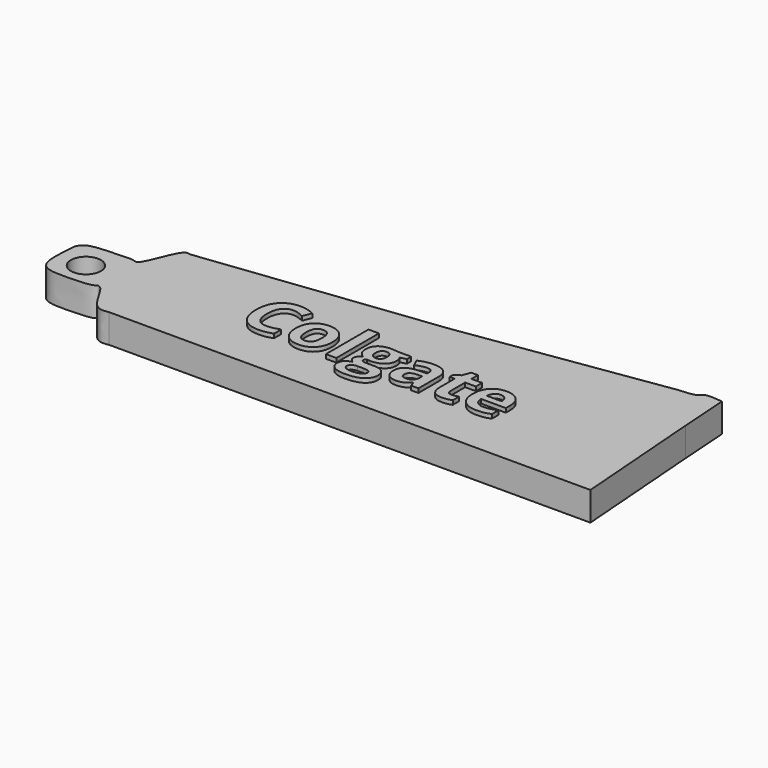
from build123d import *

# Parameters (mm, degrees)
F0_R         = 1.8236553972
F1_DEPTH     = 3.5
F2_TEXT_SIZE = 8.5194750379
F3_DEPTH     = 0.5


# Not quite as in the source:
# - Text() gives the source's letters only with a copy of the font that has no kerning and outlines rounded to 1/6400 em; it was checked with that copy


with BuildPart() as f1:
    # F0 (on Top) → F1 (new body)
    with BuildSketch(Plane.XY):
        with BuildLine():
            add(Edge.make_bspline(
                [(-94.2050293088, 31.265206635), (-94.3971896936, 31.315162363), (-94.9583376122, 31.4610433822), (-95.9054216002, 29.4777531909), (-96.8691566029, 26.8074850092), (-97.4710081074, 26.8823429315), (-97.8983149621, 27.0596648483), (-99.5300476845, 26.9187238719), (-103.2306123724, 26.9127671347), (-103.6583521932, 25.96518302), (-103.8144603372, 25.6193522364)],
                knots=[0, 0, 0, 0, 0.0806326622, 0.235463988, 0.4124921189, 0.4787807152, 0.5456222164, 0.6826832027, 0.8841918992, 1, 1, 1, 1], degree=3))
            add(Edge.make_bspline(
                [(-103.8144603372, 25.6193522364), (-103.9362776366, 24.0968857457), (-104.1299409277, 21.6764916586), (-103.0230108011, 20.2993669542), (-100.4135696071, 20.2585530739), (-97.435923479, 20.4079273263), (-97.2192654941, 20.8016425102), (-96.3493816333, 20.8286988089), (-94.7313642338, 16.8706039662), (-93.3537822149, 17.095992357), (-92.809304595, 17.1850752085)],
                knots=[0, 0, 0, 0, 0.1802033396, 0.2864845305, 0.4344172907, 0.587234469, 0.638819425, 0.7063803162, 0.883949308, 1, 1, 1, 1], degree=3))
            Line((-92.809304595, 17.1850752085), (-47.8415191174, 17.1850752085))
            Line((-47.8415191174, 17.1850752085), (-37.0270833373, 17.1850752085))
            add(Edge.make_bspline(
                [(-37.0270833373, 17.1850752085), (-36.7521914562, 17.1850752085), (-36.0885433471, 17.1850752085), (-34.9738631658, 17.1850752085), (-34.3208983541, 17.1850752085)],
                knots=[0, 0, 0, 0, 0.4142133119, 1, 1, 1, 1], degree=3))
            Line((-34.3208983541, 17.1850752085), (-35.5386808515, 33.149138093))
            Line((-35.5386808515, 33.149138093), (-35.9455570579, 39.1874983907))
            add(Edge.make_bspline(
                [(-35.9455570579, 39.1874983907), (-36.8082930393, 39.2807532353), (-38.1547953916, 39.426299347), (-38.4848889619, 38.553670295), (-39.7685209587, 38.4821076009), (-40.5851490796, 38.4365804493)],
                knots=[0, 0, 0, 0, 0.3935045367, 0.6141563534, 1, 1, 1, 1], degree=3))
            Line((-40.5851490796, 38.4365804493), (-65.6604096293, 34.6819981933))
            Line((-65.6604096293, 34.6819981933), (-94.2050293088, 31.265206635))
        make_face()
        with Locations((-100.5051881075, 23.2916418463)):
            Circle(F0_R, mode=Mode.SUBTRACT)
    extrude(amount=F1_DEPTH)

    # F2 (on face) → F3 (join)
    with BuildSketch(Plane.XY.offset(3.5)):
        with Locations((-82.1294002235, 22.5515477359)):
            Text('Colgate', F2_TEXT_SIZE, font='Open Sans', font_style=FontStyle.BOLD, text_align=(TextAlign.LEFT, TextAlign.BOTTOM))
    extrude(amount=F3_DEPTH)


solid = f1.part
